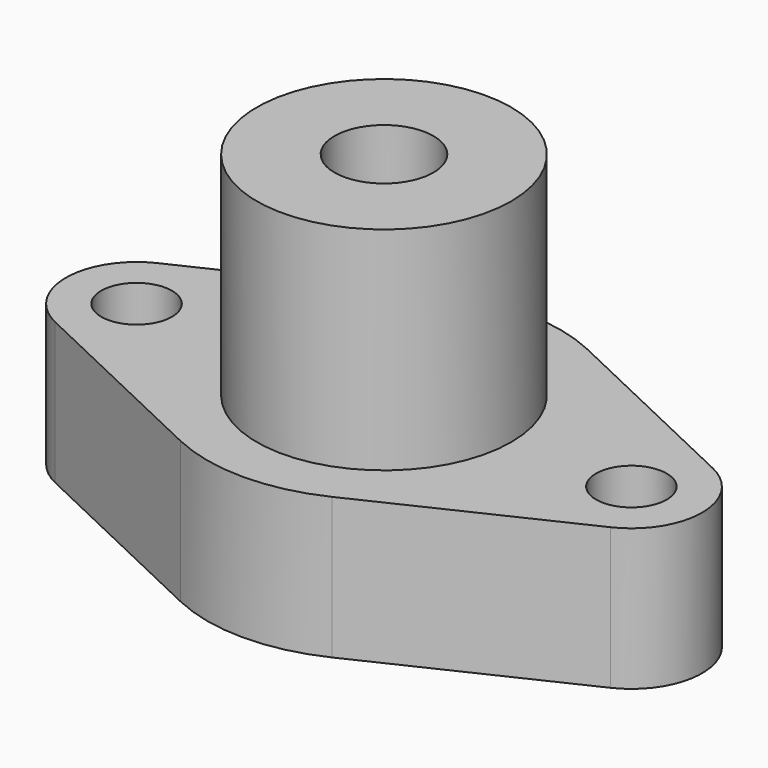
from build123d import *

# Parameters (mm, degrees)
F1_DEPTH = 20
F3_R     = 18
F4_DEPTH = 30
F6_D     = 14
F6_DEPTH = 25
F6_TIP   = 4.2060243332
F7_D     = 10


# Not quite as in the source:
# - a feature names something its author has since deleted; it is built from what else it names


with BuildPart() as f1:
    # F0 (on Top) → F1 (new body)
    with BuildSketch(Plane.XY):
        with BuildLine():
            Line((-10.7142857143, 22.5876975726), (-39.2857142857, 9.0350790291))
            ThreePointArc((-39.2857142857, 9.0350790291), (-45, 0), (-39.2857142857, -9.0350790291))
            Line((-39.2857142857, -9.0350790291), (-10.7142857143, -22.5876975726))
            ThreePointArc((-10.7142857143, -22.5876975726), (0, -25), (10.7142857143, -22.5876975726))
            Line((10.7142857143, -22.5876975726), (39.2857142857, -9.0350790291))
            ThreePointArc((39.2857142857, -9.0350790291), (45, 0), (39.2857142857, 9.0350790291))
            Line((39.2857142857, 9.0350790291), (10.7142857143, 22.5876975726))
            ThreePointArc((10.7142857143, 22.5876975726), (0, 25), (-10.7142857143, 22.5876975726))
        make_face()
    extrude(amount=-F1_DEPTH)


with BuildPart() as f1_1:
    # F2: moved
    add(f1.part.moved(Location((0, 0, 20))))

    # F3 (on face) → F4 (join)
    with BuildSketch(Plane.XY.offset(20)):
        Circle(F3_R)
    extrude(amount=F4_DEPTH)

    # F6
    with Locations(Plane.XY.offset(50)):
        with Locations((0, 0)):
            Hole(F6_D / 2, depth=F6_DEPTH)
            with Locations((0, 0, -(F6_DEPTH + F6_TIP / 2))):  # 118° drill point
                Cone(0, F6_D / 2, F6_TIP, mode=Mode.SUBTRACT)

    # F7 (through all)
    with Locations(Plane.XY.offset(20)):
        with Locations((-35, 0), (35, 0)):
            Hole(F7_D / 2)


solid = f1_1.part
